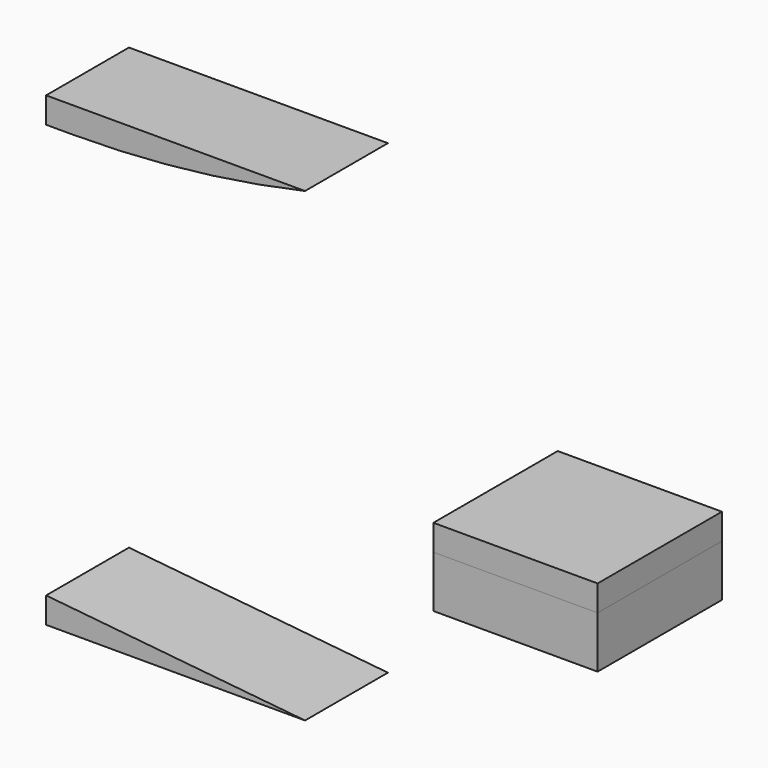
from build123d import *

# Parameters (mm, degrees)
F1_DEPTH = 10
F2_W     = 31.7073058904
F2_H     = 30
F3_DEPTH = 10
F4_DEPTH = 5


# Not quite as in the source:
# - a feature names something its author has since deleted; it is built from what else it names


with BuildPart() as f1:
    # F0 (on Front) → F1 (new body, symmetric)
    with BuildSketch(Plane.XZ):
        with BuildLine():
            Line((69.5857927203, 60), (69.5857927203, 55))
            Line((69.5857927203, 55), (74.5857927203, 55))
            ThreePointArc((74.5857927203, 55), (97.2242555657, 56.2538343919), (119.5857927203, 60))
            Line((119.5857927203, 60), (69.5857927203, 60))
        make_face()
    extrude(amount=F1_DEPTH, both=True)


with BuildPart() as f1b:
    # F0 (on Front) → F1, piece 2 (new body, symmetric)
    with BuildSketch(Plane.XZ):
        Polygon((119.5857927203, -30), (69.5857927203, -25), (69.5857927203, -30), align=None)
    extrude(amount=F1_DEPTH, both=True)


with BuildPart() as f3:
    # F2 (on Top) → F3 (new body)
    with BuildSketch(Plane.XY):
        with Locations((164.2224490643, 0)):
            Rectangle(F2_W, F2_H)
    extrude(amount=F3_DEPTH)


with BuildPart() as f4:
    # F4 (new): a face of the model
    f4_faces = [f3.part.faces().sort_by_distance(p)[0] for p in [
        (164.2224490643, 0, 10),
    ]]
    extrude(f4_faces, amount=F4_DEPTH)


solid = Compound([f1.part, f1b.part, f3.part, f4.part])
